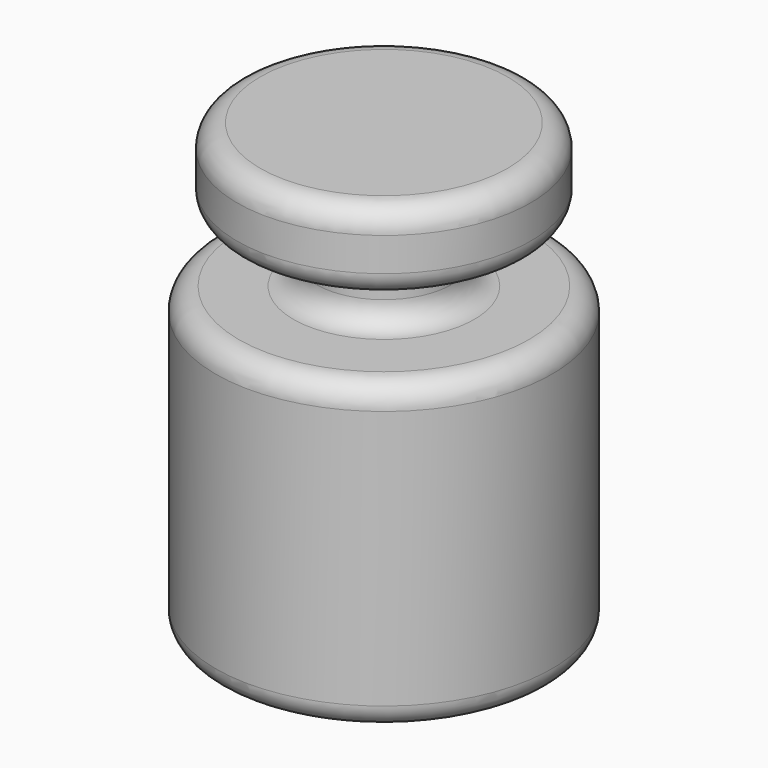
from build123d import *

# Parameters (mm, degrees)
F0_W = 5.8661173098
F0_H = 5.5776182562
F2_R = 2
F3_R = 2


# Not quite as in the source:
# - a feature of the source that left no trace in its solid (it failed there, or was rolled back) is left out


with BuildPart() as f1:
    # F0 (on Front) → F1 (revolve)
    with BuildSketch(Plane.XZ):
        Polygon((0, 35.7737019658), (0, 42.6976457238), (-12.7588799223, 42.6976457238), (-12.7588799223, 35.7737019658), (-5.8661173098, 35.7737019658), align=None)
        with Locations((-2.9330586549, 32.9848928377)):
            Rectangle(F0_W, F0_H)
        Polygon((0, 3.6543027963), (0, 30.1960837096), (-5.8661173098, 30.1960837096), (-14.617213048, 30.1960837096), (-14.617213048, 3.6543027963), align=None)
    revolve(axis=Axis((0, 0, 23.1759742601), (0, 0, -1)))

    # F2
    f2_edges = [f1.edges().sort_by_distance(p)[0] for p in [
        (12.75888, 0, 42.697646),
        (5.866117, 0, 30.196084),
        (14.617213, 0, 30.196084),
    ]]
    fillet(f2_edges, radius=F2_R)

    # F3
    f3_edges = [f1.edges().sort_by_distance(p)[0] for p in [
        (12.75888, 0, 35.773702),
        (14.617213, 0, 3.654303),
    ]]
    fillet(f3_edges, radius=F3_R)


solid = f1.part
